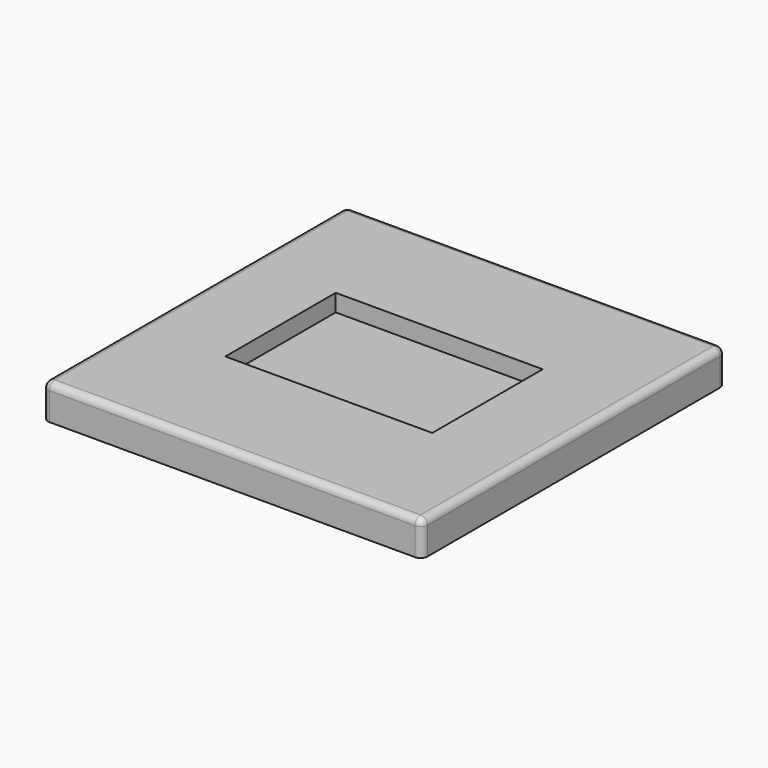
from build123d import *

# Parameters (mm, degrees)
F0_W         = 550
F0_H         = 550
F1_DEPTH     = 50
F2_R         = 10
F3_T1_DEPTH  = 65
F3_S5_W      = 10
F3_S5_H      = 10
F3_T6_DEPTH  = 10
F3_S11_W     = 10
F3_S11_H     = 10
F3_T12_DEPTH = 10
F3_S17_W     = 10
F3_S17_H     = 10
F3_T18_DEPTH = 10
F3_S23_W     = 10
F3_S23_H     = 10
F3_T24_DEPTH = 10
F4_W         = 300
F4_H         = 200
F5_DEPTH     = 25


# Not quite as in the source:
# - a fillet or chamfer that OpenCascade refuses, or shapes differently, is made with other operations: its cross-section is extruded or revolved along the edge and cut away or added


with BuildPart() as f1:
    # F0 (on Top) → F1 (new body)
    with BuildSketch(Plane.XY):
        Rectangle(F0_W, F0_H)
    extrude(amount=F1_DEPTH)

    # F2
    f2_edges = [f1.edges().sort_by_distance(p)[0] for p in [
        (0, -275, 50),
        (275, 0, 50),
        (0, 275, 50),
        (-275, 0, 50),
    ]]
    fillet(f2_edges, radius=F2_R)

    # F3: fillet of radius 10 on 4 edges, made by hand

    # F3_s2 → F3_t1 (cut)
    with BuildSketch(Plane.XY.offset(-25)):
        with BuildLine():
            ThreePointArc((275, -265), (272.0710678119, -272.0710678119), (265, -275))
            Line((265, -275), (275, -275))
            Line((275, -275), (275, -265))
        make_face()
        with BuildLine():
            ThreePointArc((-265, -275), (-272.0710678119, -272.0710678119), (-275, -265))
            Line((-275, -265), (-275, -275))
            Line((-275, -275), (-265, -275))
        make_face()
        with BuildLine():
            ThreePointArc((-265, 275), (-272.0710678119, 272.0710678119), (-275, 265))
            Line((-275, 265), (-275, 275))
            Line((-275, 275), (-265, 275))
        make_face()
        with BuildLine():
            ThreePointArc((275, 265), (272.0710678119, 272.0710678119), (265, 275))
            Line((265, 275), (275, 275))
            Line((275, 275), (275, 265))
        make_face()
    extrude(amount=F3_T1_DEPTH, mode=Mode.SUBTRACT)


with BuildPart() as f3_tool4:
    # F3_s5 → F3_t6 (new body)
    with BuildSketch(Plane.YZ.offset(265)):
        with Locations((270, 45)):
            Rectangle(F3_S5_W, F3_S5_H)
    extrude(amount=F3_T6_DEPTH)

    # F3_s7 → F3_t8 (revolve, cut)
    with BuildSketch(Plane(origin=(265, 265, 40), x_dir=(0, -0.7071067812, -0.7071067812), z_dir=(0, -0.7071067812, 0.7071067812))):
        with BuildLine():
            ThreePointArc((0, -10), (10, 0), (0, 10))
            Line((0, 10), (0, -10))
        make_face()
    revolve(axis=Axis((265, 265, 40), (1, 0, 0)), mode=Mode.SUBTRACT)


with BuildPart() as f1_1:
    add(f1.part)

    # F3_t3: cut F3_tool4
    add(f3_tool4.part, mode=Mode.SUBTRACT)


with BuildPart() as f3_tool10:
    # F3_s11 → F3_t12 (new body)
    with BuildSketch(Plane.XZ.offset(-265)):
        with Locations((-270, 45)):
            Rectangle(F3_S11_W, F3_S11_H)
    extrude(amount=-F3_T12_DEPTH)

    # F3_s13 → F3_t14 (revolve, cut)
    with BuildSketch(Plane(origin=(-265, 265, 40), x_dir=(0.7071067812, 0, -0.7071067812), z_dir=(0.7071067812, 0, 0.7071067812))):
        with BuildLine():
            ThreePointArc((0, -10), (10, 0), (0, 10))
            Line((0, 10), (0, -10))
        make_face()
    revolve(axis=Axis((-265, 265, 40), (0, 1, 0)), mode=Mode.SUBTRACT)


with BuildPart() as f1_2:
    add(f1_1.part)

    # F3_t9: cut F3_tool10
    add(f3_tool10.part, mode=Mode.SUBTRACT)


with BuildPart() as f3_tool16:
    # F3_s17 → F3_t18 (new body)
    with BuildSketch(Plane.XZ.offset(265)):
        with Locations((-270, 45)):
            Rectangle(F3_S17_W, F3_S17_H)
    extrude(amount=F3_T18_DEPTH)

    # F3_s19 → F3_t20 (revolve, cut)
    with BuildSketch(Plane(origin=(-265, -265, 40), x_dir=(0.7071067812, 0, -0.7071067812), z_dir=(-0.7071067812, 0, -0.7071067812))):
        with BuildLine():
            ThreePointArc((0, -10), (10, 0), (0, 10))
            Line((0, 10), (0, -10))
        make_face()
    revolve(axis=Axis((-265, -265, 40), (0, -1, 0)), mode=Mode.SUBTRACT)


with BuildPart() as f1_3:
    add(f1_2.part)

    # F3_t15: cut F3_tool16
    add(f3_tool16.part, mode=Mode.SUBTRACT)


with BuildPart() as f3_tool22:
    # F3_s23 → F3_t24 (new body)
    with BuildSketch(Plane.YZ.offset(265)):
        with Locations((-270, 45)):
            Rectangle(F3_S23_W, F3_S23_H)
    extrude(amount=F3_T24_DEPTH)

    # F3_s25 → F3_t26 (revolve, cut)
    with BuildSketch(Plane(origin=(265, -265, 40), x_dir=(0, 0.7071067812, -0.7071067812), z_dir=(0, -0.7071067812, -0.7071067812))):
        with BuildLine():
            ThreePointArc((0, -10), (10, 0), (0, 10))
            Line((0, 10), (0, -10))
        make_face()
    revolve(axis=Axis((265, -265, 40), (1, 0, 0)), mode=Mode.SUBTRACT)


with BuildPart() as f1_4:
    add(f1_3.part)

    # F3_t21: cut F3_tool22
    add(f3_tool22.part, mode=Mode.SUBTRACT)

    # F4 (on face) → F5 (cut)
    with BuildSketch(Plane.XY.offset(50)):
        Rectangle(F4_W, F4_H)
    extrude(amount=-F5_DEPTH, mode=Mode.SUBTRACT)


solid = f1_4.part
